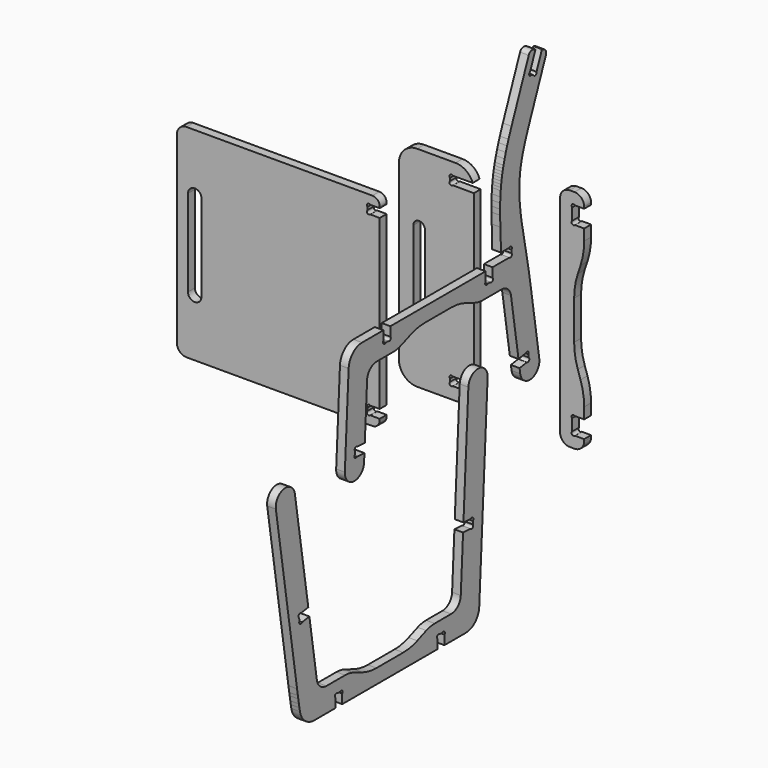
from build123d import *

# Parameters (mm, degrees)
F2_DEPTH  = 18
F4_DEPTH  = 18
F6_DEPTH  = 18
F8_DEPTH  = 18
F10_DEPTH = 18


# Not quite as in the source:
# - ends of sketch curves that miss each other by under 0.0002 mm in the source are joined


with BuildPart() as f2:
    # F1 (on Right) → F2 (new body)
    with BuildSketch(Plane.YZ):
        with BuildLine():
            Line((-83.9316420219, 195.9291984331), (-83.2733020219, 173.8269384331))
            ThreePointArc((-83.2733020219, 173.8269384331), (-82.3639869092, 150.347562221), (-81.8886271383, 126.8553934318))
            Line((-81.8886271383, 126.8553934318), (-60.1798580219, 126.8554554331))
            ThreePointArc((-60.1798580219, 126.8554554331), (-54.5230031471, 126.8554588078), (-54.5230013971, 121.1986038083))
            Line((-54.5230013971, 121.1986038083), (-54.5230010219, 114.5123274331))
            ThreePointArc((-54.5230010219, 114.5123274331), (-54.5229991471, 108.8554730583), (-60.1798536466, 108.8554718083))
            Line((-60.1798536466, 108.8554718083), (-103.5741480219, 108.8554714331))
            Line((-103.5741480219, 108.8554714331), (-103.5741480219, 89.5123274331))
            ThreePointArc((-103.5741480219, 89.5123274331), (-103.5741461471, 83.8554730583), (-109.2310006466, 83.8554718083))
            Line((-109.2310006466, 83.8554718083), (-115.9172770219, 83.8554714331))
            ThreePointArc((-115.9172770219, 83.8554714331), (-121.5741238966, 83.8554630583), (-121.5741481466, 89.5123095578))
            Line((-121.5741481466, 89.5123095578), (-121.5741480219, 108.8554714331))
            Line((-121.5741480219, 108.8554714331), (-368.7471220219, 108.8554714331))
            Line((-368.7471220219, 108.8554714331), (-368.7471220219, 89.5123124331))
            ThreePointArc((-368.7471220219, 89.5123124331), (-368.7471436471, 83.8554655583), (-374.4039901466, 83.8554713083))
            Line((-374.4039901466, 83.8554713083), (-381.0902660219, 83.8554714331))
            ThreePointArc((-381.0902660219, 83.8554714331), (-386.7471203966, 83.8554705583), (-386.7471221466, 89.5123245578))
            Line((-386.7471221466, 89.5123245578), (-386.7471220219, 108.8554714331))
            Line((-386.7471220219, 108.8554714331), (-442.0863530219, 108.8554714331))
            ThreePointArc((-442.0863530219, 108.8554714331), (-466.1711140086, 99.2508329101), (-477.0372785881, 75.7082914101))
            Line((-477.0372785881, 75.7082914101), (-486.8725900219, -109.8211165669))
            ThreePointArc((-486.8725900219, -109.8211165669), (-463.2310865178, -136.1095049897), (-436.9426985741, -112.4680015907))
            Line((-436.9426985741, -112.4680015907), (-436.0414330219, -95.4668245669))
            Line((-436.0414330219, -95.4668245669), (-455.3574240219, -94.4428085669))
            ThreePointArc((-455.3574240219, -94.4428085669), (-461.0063407033, -94.1433347301), (-460.7068761868, -88.4944173835))
            Line((-460.7068761868, -88.4944173835), (-460.3529190219, -81.8175165669))
            ThreePointArc((-460.3529190219, -81.8175165669), (-460.0534529365, -76.1685896619), (-454.4045268423, -76.4680644054))
            Line((-454.4045268423, -76.4680644054), (-435.0885520219, -77.4920325669))
            Line((-435.0885520219, -77.4920325669), (-429.1156320219, 35.1789144331))
            ThreePointArc((-429.1156320219, 35.1789144331), (-421.3540854073, 51.9950152417), (-404.1506850219, 58.8554714331))
            Line((-404.1506850219, 58.8554714331), (-361.4166740219, 58.8554714331))
            ThreePointArc((-361.4166740219, 58.8554714331), (-350.3536029427, 59.884220879), (-339.6699027038, 62.9351906151))
            Line((-339.6699027038, 62.9351906151), (-316.2166020219, 72.0559074331))
            ThreePointArc((-316.2166020219, 72.0559074331), (-298.4104285262, 77.1408586413), (-279.9719700219, 78.8554404331))
            Line((-279.9719700219, 78.8554404331), (-210.3492900219, 78.8554404331))
            ThreePointArc((-210.3492900219, 78.8554404331), (-191.9108383335, 77.140858044), (-174.1046713675, 72.0559085443))
            Line((-174.1046713675, 72.0559085443), (-150.6513690219, 62.9351914331))
            ThreePointArc((-150.6513690219, 62.9351914331), (-139.9676650685, 59.8842204976), (-128.9045900219, 58.8554714331))
            Line((-128.9045900219, 58.8554714331), (-80.3976950219, 58.8554714331))
            ThreePointArc((-80.3976950219, 58.8554714331), (-64.147811008, 52.8539249764), (-55.6998813353, 37.7307713839))
            Line((-55.6998813353, 37.7307713839), (-36.2506620219, -86.2217075669))
            Line((-36.2506620219, -86.2217075669), (-17.1413240219, -83.2232835669))
            ThreePointArc((-17.1413240219, -83.2232835669), (-11.5528479841, -82.3464015152), (-10.6759641473, -87.9348774755))
            Line((-10.6759641473, -87.9348774755), (-9.6395080219, -94.5403335669))
            ThreePointArc((-9.6395080219, -94.5403335669), (-8.7626239701, -100.1288116046), (-14.3511021887, -101.0056937958))
            Line((-14.3511021887, -101.0056937958), (-33.4604400219, -104.0041175669))
            Line((-33.4604400219, -104.0041175669), (-31.7319850219, -115.0198595669))
            ThreePointArc((-31.7319850219, -115.0198595669), (-3.158870071, -135.8423742535), (17.6636446647, -107.2692596161))
            Line((17.6636446647, -107.2692596161), (-4.3627220219, 33.1078214331))
            Line((-4.3627220219, 33.1078214331), (-10.6183430219, 70.2932004331))
            Line((-10.6183430219, 70.2932004331), (-28.3275670219, 162.8598884331))
            Line((-28.3275670219, 162.8598884331), (-29.7978660219, 172.1766284331))
            Line((-29.7978660219, 172.1766284331), (-31.0940090219, 181.5293424331))
            Line((-31.0940090219, 181.5293424331), (-32.1846970219, 190.9212304331))
            Line((-32.1846970219, 190.9212304331), (-33.0390210219, 200.3418734331))
            Line((-33.0390210219, 200.3418734331), (-33.6261670219, 209.7774434331))
            Line((-33.6261670219, 209.7774434331), (-33.9153230219, 219.2141154331))
            Line((-33.9153230219, 219.2141154331), (-33.9385250219, 223.9285444331))
            Line((-33.9385250219, 223.9285444331), (-33.8756740219, 228.6380634331))
            Line((-33.8756740219, 228.6380634331), (-33.7229190219, 233.3409454331))
            Line((-33.7229190219, 233.3409454331), (-33.4764080219, 238.0354614331))
            Line((-33.4764080219, 238.0354614331), (-33.1322890219, 242.7198834331))
            Line((-33.1322890219, 242.7198834331), (-32.6867110219, 247.3924834331))
            Line((-32.6867110219, 247.3924834331), (-32.1358220219, 252.0515324331))
            Line((-32.1358220219, 252.0515324331), (-31.4757710219, 256.6953034331))
            Line((-31.4757710219, 256.6953034331), (-30.7043690219, 261.3223604331))
            Line((-30.7043690219, 261.3223604331), (-29.8260830219, 265.9324454331))
            Line((-29.8260830219, 265.9324454331), (-28.8470430219, 270.5255924331))
            Line((-28.8470430219, 270.5255924331), (-27.7733800219, 275.1018374331))
            Line((-27.7733800219, 275.1018374331), (-26.6112240219, 279.6612154331))
            Line((-26.6112240219, 279.6612154331), (-25.3667050219, 284.2037594331))
            Line((-25.3667050219, 284.2037594331), (-22.6550990219, 293.2384894331))
            Line((-22.6550990219, 293.2384894331), (-19.6876070219, 302.2063064331))
            Line((-19.6876070219, 302.2063064331), (-16.5132680219, 311.1074884331))
            Line((-16.5132680219, 311.1074884331), (-9.7402250219, 328.7110624331))
            Line((-9.7402250219, 328.7110624331), (34.8506329781, 440.1881954331))
            ThreePointArc((34.8506329781, 440.1881954331), (34.7573160955, 447.8412958456), (29.2797717072, 453.1868697557))
            Line((29.2797717072, 453.1868697557), (24.6373999781, 455.0438254331))
            Line((24.6373999781, 455.0438254331), (10.5111209781, 419.7280764331))
            ThreePointArc((10.5111209781, 419.7280764331), (8.4102, 414.475836382), (3.1579530477, 416.5767404629))
            Line((3.1579530477, 416.5767404629), (-3.0501000219, 419.0599594331))
            ThreePointArc((-3.0501000219, 419.0599594331), (-8.3023578747, 421.1608582819), (-6.2014601989, 426.4131168463))
            Line((-6.2014601989, 426.4131168463), (7.9248139781, 461.7288534331))
            Line((7.9248139781, 461.7288534331), (3.2824579781, 463.5857954331))
            ThreePointArc((3.2824579781, 463.5857954331), (-4.3706414343, 463.4924775504), (-9.7162148617, 458.014934369))
            Line((-9.7162148617, 458.014934369), (-54.3071190219, 346.5378134331))
            Line((-54.3071190219, 346.5378134331), (-62.1610840219, 325.8800364331))
            Line((-62.1610840219, 325.8800364331), (-65.8068920219, 315.4311554331))
            Line((-65.8068920219, 315.4311554331), (-69.2113040219, 304.9032874331))
            Line((-69.2113040219, 304.9032874331), (-72.3338610219, 294.2971884331))
            Line((-72.3338610219, 294.2971884331), (-75.1341040219, 283.6136134331))
            Line((-75.1341040219, 283.6136134331), (-76.4007130219, 278.2430084331))
            Line((-76.4007130219, 278.2430084331), (-77.5715730219, 272.8533184331))
            Line((-77.5715730219, 272.8533184331), (-78.6416230219, 267.4446374331))
            Line((-78.6416230219, 267.4446374331), (-79.6058090219, 262.0170604331))
            Line((-79.6058090219, 262.0170604331), (-80.4607220219, 256.5709604331))
            Line((-80.4607220219, 256.5709604331), (-81.2095660219, 251.1078284331))
            Line((-81.2095660219, 251.1078284331), (-81.8571910219, 245.6294354331))
            Line((-81.8571910219, 245.6294354331), (-82.4084500219, 240.1375504331))
            Line((-82.4084500219, 240.1375504331), (-83.2412800219, 229.1203864331))
            Line((-83.2412800219, 229.1203864331), (-83.7468760219, 218.0704994331))
            Line((-83.7468760219, 218.0704994331), (-83.9640570219, 207.0020494331))
            Line((-83.9640570219, 207.0020494331), (-83.9316420219, 195.9291984331))
        make_face()
    extrude(amount=F2_DEPTH)


with BuildPart() as f4:
    # F3 (on Right) → F4 (new body)
    with BuildSketch(Plane.YZ):
        with BuildLine():
            ThreePointArc((-186.0517315499, -457.4372610121), (-193.8132765435, -474.2533617835), (-211.0166759977, -481.1138189884))
            Line((-211.0166759977, -481.1138189884), (-253.7505609977, -481.1138189884))
            ThreePointArc((-253.7505609977, -481.1138189884), (-264.8136358662, -482.1425680195), (-275.4973397152, -485.1935387147))
            Line((-275.4973397152, -485.1935387147), (-298.9507639977, -494.3142869884))
            ThreePointArc((-298.9507639977, -494.3142869884), (-316.7569311311, -499.3992365659), (-335.1953829977, -501.1138189884))
            Line((-335.1953829977, -501.1138189884), (-404.8179409977, -501.1138189884))
            ThreePointArc((-404.8179409977, -501.1138189884), (-423.2563996802, -499.3992371632), (-441.0625732713, -494.3142856921))
            Line((-441.0625732713, -494.3142856921), (-464.5159969977, -485.1935379884))
            ThreePointArc((-464.5159969977, -485.1935379884), (-475.1996970966, -482.1425684008), (-486.2627679977, -481.1138189884))
            Line((-486.2627679977, -481.1138189884), (-534.7696049977, -481.1138189884))
            ThreePointArc((-534.7696049977, -481.1138189884), (-551.0194902516, -475.1122731817), (-559.4674206842, -459.9891189392))
            Line((-559.4674206842, -459.9891189392), (-578.9167009977, -336.0366399884))
            Line((-578.9167009977, -336.0366399884), (-598.0259779977, -339.0350489884))
            ThreePointArc((-598.0259779977, -339.0350489884), (-603.6144426076, -339.9119386393), (-604.4913524173, -334.3234764113))
            Line((-604.4913524173, -334.3234764113), (-605.5278329977, -327.7180039884))
            ThreePointArc((-605.5278329977, -327.7180039884), (-606.4047486486, -322.1295193784), (-600.8162599195, -321.2526288811))
            Line((-600.8162599195, -321.2526288811), (-581.7068619977, -318.2542149884))
            Line((-581.7068619977, -318.2542149884), (-616.4334859977, -96.9363339884))
            ThreePointArc((-616.4334859977, -96.9363339884), (-645.0066009485, -76.1138193018), (-665.8291156842, -104.6869339392))
            Line((-665.8291156842, -104.6869339392), (-610.8045189977, -455.3661839884))
            Line((-610.8045189977, -455.3661839884), (-608.7246849977, -468.5163309884))
            Line((-608.7246849977, -468.5163309884), (-607.6542499977, -475.1069379884))
            Line((-607.6542499977, -475.1069379884), (-605.9872579977, -485.0257759884))
            Line((-605.9872579977, -485.0257759884), (-604.6800069977, -492.4970739884))
            Line((-604.6800069977, -492.4970739884), (-603.3205389977, -499.9998509884))
            ThreePointArc((-603.3205389977, -499.9998509884), (-590.263552244, -522.3171517405), (-565.9496579977, -531.1138189884))
            Line((-565.9496579977, -531.1138189884), (-511.5932149977, -531.1138189884))
            Line((-511.5932149977, -531.1138189884), (-511.5932149977, -511.7706729884))
            ThreePointArc((-511.5932149977, -511.7706729884), (-511.5932151224, -506.1138188636), (-505.9363608729, -506.1138188636))
            Line((-505.9363608729, -506.1138188636), (-499.2500689977, -506.1138189884))
            ThreePointArc((-499.2500689977, -506.1138189884), (-493.5932148729, -506.1138188636), (-493.5932148729, -511.7706731131))
            Line((-493.5932148729, -511.7706731131), (-493.5932149977, -531.1138189884))
            Line((-493.5932149977, -531.1138189884), (-246.4201189977, -531.1138189884))
            Line((-246.4201189977, -531.1138189884), (-246.4201189977, -511.7706729884))
            ThreePointArc((-246.4201189977, -511.7706729884), (-246.4201191224, -506.1138188636), (-240.7632648729, -506.1138188636))
            Line((-240.7632648729, -506.1138188636), (-234.0769729977, -506.1138189884))
            ThreePointArc((-234.0769729977, -506.1138189884), (-228.4201188729, -506.1138188636), (-228.4201188729, -511.7706731131))
            Line((-228.4201188729, -511.7706731131), (-228.4201189977, -531.1138189884))
            Line((-228.4201189977, -531.1138189884), (-173.0810059977, -531.1138189884))
            ThreePointArc((-173.0810059977, -531.1138189884), (-148.9962472166, -521.5091787638), (-138.1300843814, -497.9666380211))
            Line((-138.1300843814, -497.9666380211), (-116.3652079977, -87.4021969884))
            ThreePointArc((-116.3652079977, -87.4021969884), (-140.0067105017, -61.1138095657), (-166.2950983954, -84.7553120203))
            Line((-166.2950983954, -84.7553120203), (-179.1259299977, -326.7915379884))
            Line((-179.1259299977, -326.7915379884), (-159.5029249977, -327.8317909884))
            ThreePointArc((-159.5029249977, -327.8317909884), (-153.8777754162, -328.4298729226), (-154.4758587814, -334.0550222561))
            Line((-154.4758587814, -334.0550222561), (-154.8143839977, -340.4408199884))
            ThreePointArc((-154.8143839977, -340.4408199884), (-155.1138456342, -346.0897408925), (-160.762767181, -345.7902801533))
            Line((-160.762767181, -345.7902801533), (-180.0788109977, -344.7662999884))
            Line((-180.0788109977, -344.7662999884), (-186.0517315499, -457.4372610121))
        make_face()
    extrude(amount=F4_DEPTH)


with BuildPart() as f6:
    # F5 (on Front) → F6 (new body)
    with BuildSketch(Plane.XZ):
        with BuildLine():
            ThreePointArc((-127.3587303294, -217.5000011921), (-105.564234066, -210.6287663427), (-91.6515858819, -192.500000355))
            Line((-91.6515858819, -192.500000355), (-133.0919493294, -192.3000011921))
            ThreePointArc((-133.0919493294, -192.3000011921), (-138.7488037041, -192.3000000668), (-138.7488034541, -186.6431460673))
            Line((-138.7488034541, -186.6431460673), (-138.7488033294, -180.3568551921))
            ThreePointArc((-138.7488033294, -180.3568551921), (-138.7488034541, -174.7000010673), (-133.0919492046, -174.7000010673))
            Line((-133.0919492046, -174.7000010673), (-89.3587283294, -174.5000011921))
            Line((-89.3587283294, -174.5000011921), (-89.3587283294, 174.5000058079))
            Line((-89.3587283294, 174.5000058079), (-133.0919493294, 174.7000058079))
            ThreePointArc((-133.0919493294, 174.7000058079), (-138.7488037041, 174.7000069332), (-138.7488034541, 180.3568609327))
            Line((-138.7488034541, 180.3568609327), (-138.7488033294, 186.6431518079))
            ThreePointArc((-138.7488033294, 186.6431518079), (-138.7488034541, 192.3000059327), (-133.0919492046, 192.3000059327))
            Line((-133.0919492046, 192.3000059327), (-91.6515863294, 192.5000058079))
            ThreePointArc((-91.6515863294, 192.5000058079), (-105.5642344508, 210.628771228), (-127.3587303294, 217.5000058079))
            Line((-127.3587303294, 217.5000058079), (-206.9417983294, 217.5000058079))
            ThreePointArc((-206.9417983294, 217.5000058079), (-233.8118557822, 206.3700617252), (-244.9417963294, 179.5000028079))
            Line((-244.9417963294, 179.5000028079), (-244.9417963294, -179.4999971921))
            ThreePointArc((-244.9417963294, -179.4999971921), (-233.8118561358, -206.3700567559), (-206.9417983294, -217.5000011921))
            Line((-206.9417983294, -217.5000011921), (-127.3587303294, -217.5000011921))
        make_face()
        with BuildLine():
            ThreePointArc((-190.9417963294, -75.0000011921), (-202.9417958294, -87.0000011921), (-214.9417963294, -75.0000021921))
            Line((-214.9417963294, -75.0000021921), (-214.9417963294, 75.0000048079))
            ThreePointArc((-214.9417963294, 75.0000048079), (-202.9417968294, 87.0000058079), (-190.9417963294, 75.0000058079))
            Line((-190.9417963294, 75.0000058079), (-190.9417963294, -75.0000011921))
        make_face(mode=Mode.SUBTRACT)
    extrude(amount=F6_DEPTH)


with BuildPart() as f8:
    # F7 (on Front) → F8 (new body)
    with BuildSketch(Plane.XZ):
        with BuildLine():
            Line((109.7173344402, -224.4963243451), (119.7173344402, -224.4963243451))
            ThreePointArc((119.7173344402, -224.4963243451), (133.8594707104, -218.6384603224), (139.7173354402, -204.4963243451))
            Line((139.7173354402, -204.4963243451), (139.7173354402, -200.4963243451))
            Line((139.7173354402, -200.4963243451), (120.3741894402, -200.4963243451))
            ThreePointArc((120.3741894402, -200.4963243451), (114.7173350655, -200.4963232199), (114.7173353155, -194.8394692204))
            Line((114.7173353155, -194.8394692204), (114.7173354402, -170.1531783451))
            ThreePointArc((114.7173354402, -170.1531783451), (114.7173353155, -164.4963242204), (120.374189565, -164.4963242204))
            Line((120.374189565, -164.4963242204), (139.7173354402, -164.4963243451))
            Line((139.7173354402, -164.4963243451), (139.7173354402, -141.5277123451))
            ThreePointArc((139.7173354402, -141.5277123451), (137.8120554999, -117.6959291459), (132.1446169008, -94.4695621929))
            Line((132.1446169008, -94.4695621929), (126.5058734402, -77.4030773451))
            ThreePointArc((126.5058734402, -77.4030773451), (120.8384342435, -54.1767034784), (118.9331554402, -30.3449133451))
            Line((118.9331554402, -30.3449133451), (118.9331554402, 50.3522646549))
            ThreePointArc((118.9331554402, 50.3522646549), (120.8384343229, 74.1840542818), (126.5058738812, 97.4104275092))
            Line((126.5058738812, 97.4104275092), (132.1446164402, 114.4769276549))
            ThreePointArc((132.1446164402, 114.4769276549), (137.8120554999, 137.7032944556), (139.7173354402, 161.5350776549))
            Line((139.7173354402, 161.5350776549), (139.7173354402, 184.5037056549))
            Line((139.7173354402, 184.5037056549), (120.3741894402, 184.5037056549))
            ThreePointArc((120.3741894402, 184.5037056549), (114.7173350655, 184.5037067801), (114.7173353155, 190.1605607796))
            Line((114.7173353155, 190.1605607796), (114.7173354402, 214.8468516549))
            ThreePointArc((114.7173354402, 214.8468516549), (114.7173353155, 220.5037057796), (120.374189565, 220.5037057796))
            Line((120.374189565, 220.5037057796), (139.7173354402, 220.5037056549))
            Line((139.7173354402, 220.5037056549), (139.7173354402, 224.5037056549))
            ThreePointArc((139.7173354402, 224.5037056549), (133.8594707104, 238.6458416322), (119.7173344402, 244.5037056549))
            Line((119.7173344402, 244.5037056549), (109.7173344402, 244.5037056549))
            ThreePointArc((109.7173344402, 244.5037056549), (95.5751991094, 238.6458405715), (89.7173354402, 224.5037046549))
            Line((89.7173354402, 224.5037046549), (89.7173354402, -204.4963253451))
            ThreePointArc((89.7173354402, -204.4963253451), (95.5751998165, -218.6384599689), (109.7173344402, -224.4963243451))
        make_face()
    extrude(amount=F8_DEPTH)


with BuildPart() as f10:
    # F9 (on Front) → F10 (new body)
    with BuildSketch(Plane.XZ):
        with BuildLine():
            ThreePointArc((-299.7393172846, -319.3985521793), (-289.1327149204, -315.0051542507), (-284.7393162846, -304.3985521793))
            Line((-284.7393162846, -304.3985521793), (-284.7393162846, -301.3985521793))
            Line((-284.7393162846, -301.3985521793), (-304.5187412846, -301.1985521793))
            ThreePointArc((-304.5187412846, -301.1985521793), (-310.1755956594, -301.1985510541), (-310.1755954094, -295.5416970546))
            Line((-310.1755954094, -295.5416970546), (-310.1755952846, -289.2554061793))
            ThreePointArc((-310.1755952846, -289.2554061793), (-310.1755954094, -283.5985520546), (-304.5187411599, -283.5985520546))
            Line((-304.5187411599, -283.5985520546), (-284.7393162846, -283.3985521793))
            Line((-284.7393162846, -283.3985521793), (-284.7393162846, 65.6014478207))
            Line((-284.7393162846, 65.6014478207), (-304.5187412846, 65.8014478207))
            ThreePointArc((-304.5187412846, 65.8014478207), (-310.1755956594, 65.8014489459), (-310.1755954094, 71.4583029454))
            Line((-310.1755954094, 71.4583029454), (-310.1755952846, 77.7445938207))
            ThreePointArc((-310.1755952846, 77.7445938207), (-310.1755954094, 83.4014479454), (-304.5187411599, 83.4014479454))
            Line((-304.5187411599, 83.4014479454), (-284.7393162846, 83.6014478207))
            Line((-284.7393162846, 83.6014478207), (-284.7393162846, 86.6014478207))
            ThreePointArc((-284.7393162846, 86.6014478207), (-289.1327149204, 97.208049892), (-299.7393172846, 101.6014478207))
            Line((-299.7393172846, 101.6014478207), (-685.7122182846, 101.6014478207))
            ThreePointArc((-685.7122182846, 101.6014478207), (-699.8543536154, 95.7435827373), (-705.7122172846, 81.6014468207))
            Line((-705.7122172846, 81.6014468207), (-705.7122172846, -299.3985531793))
            ThreePointArc((-705.7122172846, -299.3985531793), (-699.8543529083, -313.5406878031), (-685.7122182846, -319.3985521793))
            Line((-685.7122182846, -319.3985521793), (-299.7393172846, -319.3985521793))
        make_face()
        with BuildLine():
            Line((-682.7122172846, -198.8985531793), (-682.7122172846, -18.8985501793))
            ThreePointArc((-682.7122172846, -18.8985501793), (-668.7122162846, -4.8985521793), (-654.7122172846, -18.8985521793))
            Line((-654.7122172846, -18.8985521793), (-654.7122172846, -198.8985521793))
            ThreePointArc((-654.7122172846, -198.8985521793), (-668.7122167846, -212.8985521793), (-682.7122172846, -198.8985531793))
        make_face(mode=Mode.SUBTRACT)
    extrude(amount=F10_DEPTH)


solid = Compound([f2.part, f4.part, f6.part, f8.part, f10.part])
